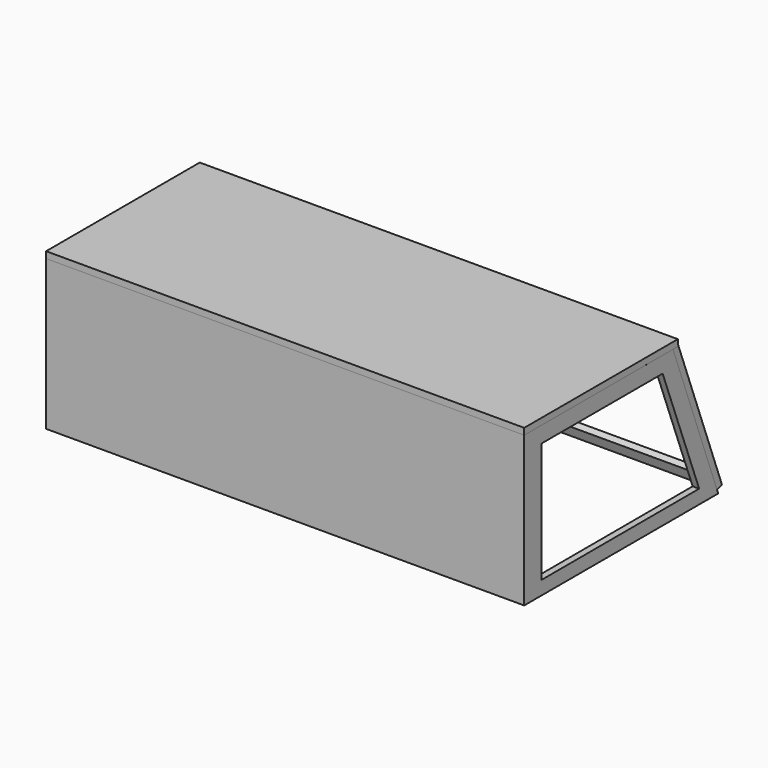
from build123d import *

# Parameters (mm, degrees)
F1_DEPTH  = 0.55
F2_W      = 78.9
F2_H      = 25.4280829926
F2_W_2    = 1.1
F3_DEPTH  = 1.1
F4_W      = 1.1
F4_H      = 25.4280829926
F5_DEPTH  = 1.1
F6_W      = 78.9
F6_H      = 26.5003892772
F6_W_2    = 76.2348438147
F6_H_2    = 22.5544893183
F6_W_3    = 1.1
F7_DEPTH  = 1.1
F8_DEPTH  = 1.1
F10_DEPTH = 1.1


# Not quite as in the source:
# - ends of sketch curves that miss each other by under 0.0002 mm in the source are joined
# - a feature names something its author has since deleted; it is built from what else it names


with BuildPart() as f1:
    # F0 (on Right) → F1 (new body, symmetric)
    with BuildSketch(Plane.YZ):
        Polygon((-20, 25.4280829926), (-20, 0), (-0.7378033123, 0), (0, 0), (20, 0), (10.4452063715, 25.4280829926), align=None)
        Polygon((8.2472184154, 22.693965584), (15.9812862531, 2.3275862914), (-17.4568928778, 2.3275862914), (-17.4568928778, 22.693965584), align=None, mode=Mode.SUBTRACT)
    extrude(amount=F1_DEPTH, both=True)

    # F2 (on face) → F3 (join)
    with BuildSketch(Plane.XZ.offset(20)):
        with Locations((40, 12.7140414963)):
            Rectangle(F2_W, F2_H)
        with Locations((0, 12.7140414963)):
            Rectangle(F2_W_2, F2_H)
    extrude(amount=F3_DEPTH)

    # F4 (on face) → F5 (join)
    with BuildSketch(Plane.YZ.offset(79.45)):
        Polygon((-20, 25.4280829926), (-20, 0), (0, 0), (20.0266968459, 0), (10.4452678934, 25.4279654473), align=None)
        Polygon((8.2472153008, 22.6938780397), (15.9903429449, 2.3578198161), (-17.4568258226, 2.3277304135), (-17.4568258226, 22.6938780397), align=None, mode=Mode.SUBTRACT)
        with Locations((-20.55, 12.7140414963)):
            Rectangle(F4_W, F4_H)
    extrude(amount=F5_DEPTH)

    # F6 (on face) → F7 (join)
    with BuildSketch(Plane(origin=(0, 17.5367681908, 6.6079725814), x_dir=(-1, 0, 0), z_dir=(0, 0.9357721565, 0.3526052626))):
        with Locations((-40, 6.8615309945)):
            Rectangle(F6_W, F6_H)
        with Locations((-40.4041948495, 6.8278673571)):
            Rectangle(F6_W_2, F6_H_2, mode=Mode.SUBTRACT)
        with Locations((-80, 6.8615309945)):
            Rectangle(F6_W_3, F6_H)
    extrude(amount=F7_DEPTH)


with BuildPart() as f8:
    # F6 (on face) → F8 (new body)
    with BuildSketch(Plane(origin=(0, 17.5367681908, 6.6079725814), x_dir=(-1, 0, 0), z_dir=(0, 0.9357721565, 0.3526052626))):
        with Locations((-80, 6.8615309945)):
            Rectangle(F6_W_3, F6_H)
    extrude(amount=F8_DEPTH)


with BuildPart() as f10:
    # F9 (on face) → F10 (new body)
    with BuildSketch(Plane.XY.offset(25.4280829926)):
        Polygon((79.45, -20), (80.55, -20), (80.55, 11.4747500047), (-0.55, 11.4747500047), (-0.55, 10.4452063715), (0.55, 10.4452063715), (0.55, -20), align=None)
        Polygon((-0.55, -21.1), (80.55, -21.1), (80.55, -20), (79.45, -20), (0.55, -20), (0.55, 10.4452063715), (-0.55, 10.4452063715), align=None)
    extrude(amount=F10_DEPTH)


solid = Compound([f1.part, f8.part, f10.part])
